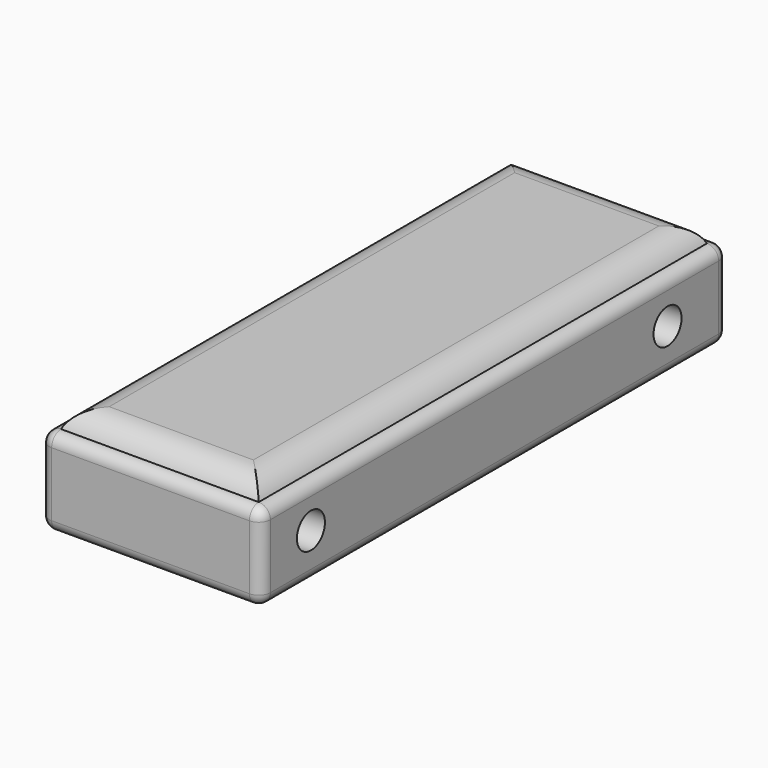
from build123d import *

# Parameters (mm, degrees)
F0_W        = 37.869092077
F0_H        = 99.9836400151
F0_W_2      = 29.556363821
F0_H_2      = 88.9000073075
F1_DEPTH    = 15
F2_R        = 2
F3_W        = 33.869092077
F3_H        = 95.9836400151
F4_DEPTH    = 3
F6_D        = 6
F7_T1_DEPTH = 56.7819705518
F7_T3_DEPTH = 118.8965184899


# Not quite as in the source:
# - a fillet or chamfer that OpenCascade refuses, or shapes differently, is made with other operations: its cross-section is extruded or revolved along the edge and cut away or added


with BuildPart() as f1:
    # F0 (on Top) → F1 (new body)
    with BuildSketch(Plane.XY):
        Rectangle(F0_W, F0_H)
        Rectangle(F0_W_2, F0_H_2, mode=Mode.SUBTRACT)
    extrude(amount=F1_DEPTH)

    # F2
    f2_edges = [f1.edges().sort_by_distance(p)[0] for p in [
        (0, 49.99182, 15),
        (-18.934546, 0, 15),
        (0, -49.99182, 15),
        (18.934546, 0, 15),
        (-18.934546, 49.99182, 7.5),
        (-18.934546, -49.99182, 7.5),
        (18.934546, 49.99182, 7.5),
        (18.934546, -49.99182, 7.5),
        (14.778182, 0, 15),
        (-14.778182, 0, 15),
        (0, -44.450004, 15),
        (0, 44.450004, 15),
        (0, -44.450004, 0),
        (0, -49.99182, 0),
        (-14.778182, 0, 0),
        (18.934546, 0, 0),
        (14.778182, 0, 0),
        (0, 44.450004, 0),
        (0, 49.99182, 0),
        (-18.934546, 0, 0),
    ]]
    fillet(f2_edges, radius=F2_R)

    # F3 (on face) → F4 (join)
    with BuildSketch(Plane.XY.offset(15)):
        Rectangle(F3_W, F3_H)
    extrude(amount=F4_DEPTH)

    # F6 (through all)
    with Locations(Plane.YZ.offset(18.9345460385)):
        with Locations((-39.3181852996, 7.8409090638), (37.0454601943, 7.6136365533)):
            Hole(F6_D / 2)

    # F7: fillet of radius 5 on 4 edges, made by hand

    # F7_s2 → F7_t1 (cut)
    with BuildSketch(Plane.YZ.offset(-28.3909852759)):
        with BuildLine():
            ThreePointArc((-43.4092443126, 18), (-46.1478571001, 17.1833001327), (-47.9918200076, 15))
            Line((-47.9918200076, 15), (-47.9918200076, 18))
            Line((-47.9918200076, 18), (-43.4092443126, 18))
        make_face()
        with BuildLine():
            ThreePointArc((47.9918200076, 15), (46.1478571001, 17.1833001327), (43.4092443126, 18))
            Line((43.4092443126, 18), (47.9918200076, 18))
            Line((47.9918200076, 18), (47.9918200076, 15))
        make_face()
    extrude(amount=F7_T1_DEPTH, mode=Mode.SUBTRACT)

    # F7_s4 → F7_t3 (cut)
    with BuildSketch(Plane.XZ.offset(-59.448259245)):
        with BuildLine():
            ThreePointArc((16.9345460385, 15), (15.0905831311, 17.1833001327), (12.3519703436, 18))
            Line((12.3519703436, 18), (16.9345460385, 18))
            Line((16.9345460385, 18), (16.9345460385, 15))
        make_face()
        with BuildLine():
            ThreePointArc((-16.9345460385, 15), (-15.0905831311, 17.1833001327), (-12.3519703436, 18))
            Line((-12.3519703436, 18), (-16.9345460385, 18))
            Line((-16.9345460385, 18), (-16.9345460385, 15))
        make_face()
    extrude(amount=F7_T3_DEPTH, mode=Mode.SUBTRACT)


solid = f1.part
